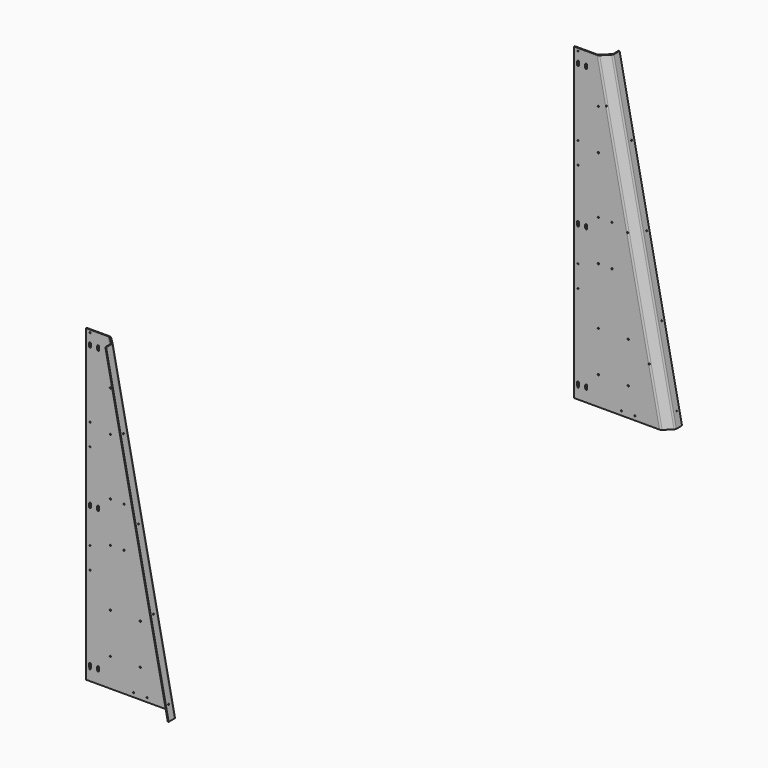
from build123d import *

# Parameters (mm, degrees)
F1_DEPTH  = 60
F2_T      = -3
F3_SIZE   = 30
F4_R      = 10
F6_R      = 2.5
F7_DEPTH  = 25
F8_D      = 4.1
F8_DEPTH  = 5
F8_TIP    = 1.231764269
F10_DEPTH = 25
F12_R     = 2.05
F13_DEPTH = 25


with BuildPart() as f1:
    # F0 (on Front) → F1 (new body)
    with BuildSketch(Plane.XZ):
        Polygon((0, 1140), (0, 0), (350, 0), (120, 1140), align=None)
    extrude(amount=-F1_DEPTH)

    # F2
    f2_openings = [f1.faces().sort_by_distance(p)[0] for p in [
        (60, 30, 1140),
        (0, 30, 570),
        (126.879433, 60, 477.021277),
        (175, 30, 0),
    ]]
    offset(amount=F2_T, openings=f2_openings)

    # F3
    f3_edges = [f1.edges().sort_by_distance(p)[0] for p in [
        (235, 0, 570),
        (231.939552, 3, 570),
    ]]
    chamfer(f3_edges, length=F3_SIZE)

    # F4
    f4_edges = [f1.edges().sort_by_distance(p)[0] for p in [
        (204.395518, 0, 570),
        (235, 30, 570),
        (201.335069, 3, 570),
        (231.939552, 33, 570),
    ]]
    fillet(f4_edges, radius=F4_R)

    # F6 (on face) → F7 (cut)
    with BuildSketch(Plane.XZ):
        with Locations((90, 105)):
            Circle(F6_R)
        with Locations((200, 105)):
            Circle(F6_R)
        with Locations((200, 255)):
            Circle(F6_R)
        with Locations((90, 255)):
            Circle(F6_R)
        with Locations((90, 465)):
            Circle(F6_R)
        with Locations((90, 615)):
            Circle(F6_R)
        with Locations((140, 465)):
            Circle(F6_R)
        with Locations((140, 615)):
            Circle(F6_R)
        with Locations((90, 825)):
            Circle(F6_R)
        with Locations((90, 975)):
            Circle(F6_R)
        with Locations((225, 15)):
            Circle(F6_R)
        with Locations((175, 15)):
            Circle(F6_R)
    extrude(amount=-F7_DEPTH, mode=Mode.SUBTRACT)

    # F8
    with Locations(Plane(origin=(336.3105360444, 0, 67.8521256932), x_dir=(0, 1, 0), z_dir=(0.9802485633, 0, 0.197769447))):
        with Locations((48, -19.2193064432), (48, 260.7806935568), (48, 540.7806935568), (48, 820.7806935568), (48, 1100.7806935568)):
            Hole(F8_D / 2, depth=F8_DEPTH)
            with Locations((0, 0, -(F8_DEPTH + F8_TIP / 2))):  # 118° drill point
                Cone(0, F8_D / 2, F8_TIP, mode=Mode.SUBTRACT)

    # F9 (on face) → F10 (cut)
    with BuildSketch(Plane.XZ):
        with BuildLine():
            ThreePointArc((11.5, 44.5), (15, 41), (18.5, 44.5))
            Line((18.5, 44.5), (18.5, 55.5))
            ThreePointArc((18.5, 55.5), (15, 59), (11.5, 55.5))
            Line((11.5, 55.5), (11.5, 44.5))
        make_face()
        with BuildLine():
            ThreePointArc((41.5, 44.5), (45, 41), (48.5, 44.5))
            Line((48.5, 44.5), (48.5, 55.5))
            ThreePointArc((48.5, 55.5), (45, 59), (41.5, 55.5))
            Line((41.5, 55.5), (41.5, 44.5))
        make_face()
        with BuildLine():
            ThreePointArc((48.5, 575.5), (45, 579), (41.5, 575.5))
            Line((41.5, 575.5), (41.5, 564.5))
            ThreePointArc((41.5, 564.5), (45, 561), (48.5, 564.5))
            Line((48.5, 564.5), (48.5, 575.5))
        make_face()
        with BuildLine():
            Line((11.5, 575.5), (11.5, 564.5))
            ThreePointArc((11.5, 564.5), (15, 561), (18.5, 564.5))
            Line((18.5, 564.5), (18.5, 575.5))
            ThreePointArc((18.5, 575.5), (15, 579), (11.5, 575.5))
        make_face()
        with BuildLine():
            ThreePointArc((48.5, 1095.5), (45, 1099), (41.5, 1095.5))
            Line((41.5, 1095.5), (41.5, 1084.5))
            ThreePointArc((41.5, 1084.5), (45, 1081), (48.5, 1084.5))
            Line((48.5, 1084.5), (48.5, 1095.5))
        make_face()
        with BuildLine():
            Line((11.5, 1095.5), (11.5, 1084.5))
            ThreePointArc((11.5, 1084.5), (15, 1081), (18.5, 1084.5))
            Line((18.5, 1084.5), (18.5, 1095.5))
            ThreePointArc((18.5, 1095.5), (15, 1099), (11.5, 1095.5))
        make_face()
    extrude(amount=-F10_DEPTH, mode=Mode.SUBTRACT)

    # F12 (on face) → F13 (cut)
    with BuildSketch(Plane.XZ):
        with Locations((15, 40)):
            Circle(F12_R)
        with Locations((277, 200)):
            Circle(F12_R)
        with Locations((15, 360)):
            Circle(F12_R)
        with Locations((15, 440)):
            Circle(F12_R)
        with Locations((15, 760)):
            Circle(F12_R)
        with Locations((15, 840)):
            Circle(F12_R)
        with Locations((15, 1130)):
            Circle(F12_R)
        with Locations((197, 600)):
            Circle(F12_R)
        with Locations((119, 985)):
            Circle(F12_R)
    extrude(amount=-F13_DEPTH, mode=Mode.SUBTRACT)


with BuildPart() as f14_1:
    # F14: instance of F1
    add(f1.part.mirror(Plane.XZ.offset(1122)))


solid = Compound([f1.part, f14_1.part])
